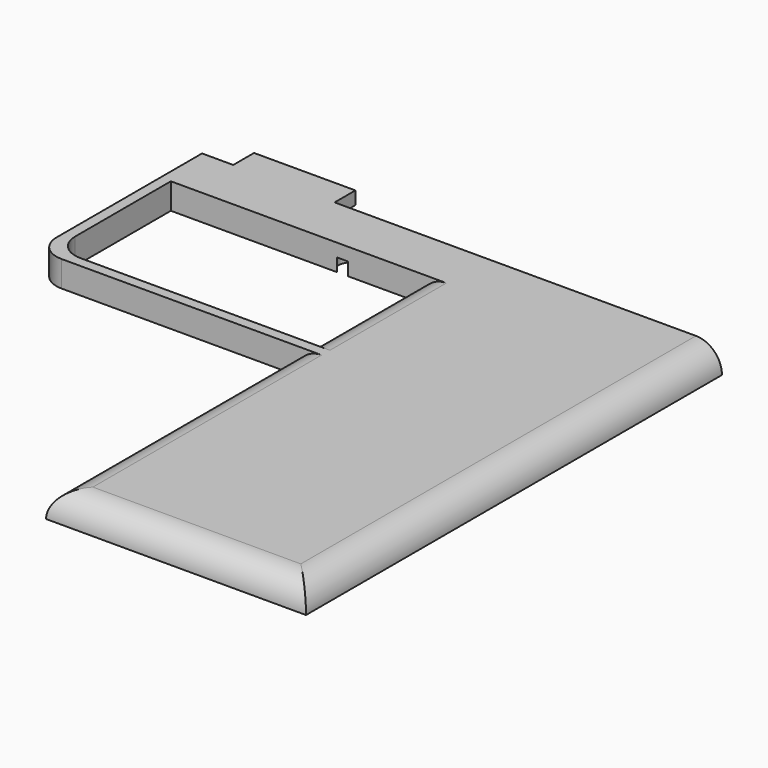
from build123d import *

# Parameters (mm, degrees)
F0_W     = 48
F0_H     = 10
F1_DEPTH = 5
F2_R     = 4.99999
F3_R     = 5
F4_W     = 6
F4_H     = 81
F4_R     = 1.75
F5_DEPTH = 2.5
F6_W     = 19.5
F6_H     = 2.5
F7_DEPTH = 5


# Not quite as in the source:
# - a fillet or chamfer is up to 0.001 mm smaller than in the source, because OpenCascade refuses the exact size


with BuildPart() as f1:
    # F0 (on Top) → F1 (new body)
    with BuildSketch(Plane.XY):
        Polygon((-73, 40), (-73, 50), (-75, 50), (-75, 10), (-25, 10), (-25, 12), (-73, 12), align=None)
        Polygon((25, -50), (25, 50), (-25, 50), (-25, 40), (-25, 12), (-25, 10), (-25, -50), align=None)
        with Locations((-49, 45)):
            Rectangle(F0_W, F0_H)
    extrude(amount=-F1_DEPTH)

    # F2 (radius 5 in the source; OpenCascade refuses exactly that, so slightly less here)
    f2_edges = [f1.edges().sort_by_distance(p)[0] for p in [
        (-25, -20, 0),
        (0, -50, 0),
        (25, 0, 0),
        (-25, 26, 0),
    ]]
    fillet(f2_edges, radius=F2_R)

    # F3
    f3_edges = [f1.edges().sort_by_distance(p)[0] for p in [
        (-73, 12, -2.5),
        (-75, 10, -2.5),
    ]]
    fillet(f3_edges, radius=F3_R)

    # F4 (on face) → F5 (cut)
    with BuildSketch(Plane(origin=(0, 0, -5), x_dir=(1, 0, 0), z_dir=(0, 0, -1))):
        Rectangle(F4_W, F4_H)
        with BuildLine():
            ThreePointArc((-41.0307764064, -40), (-41.1711646096, -43.9211646096), (-37.75, -42))
            ThreePointArc((-37.75, -42), (-38.0788353904, -40.8288353904), (-38.9692235936, -40))
            Line((-38.9692235936, -40), (-41.0307764064, -40))
        make_face()
        with Locations((-50, -48)):
            Circle(F4_R)
        with Locations((-62.5, -45)):
            Circle(F4_R)
        with BuildLine():
            ThreePointArc((-71.25, -42), (-71.7625631329, -40.7625631329), (-73, -40.25))
            ThreePointArc((-73, -40.25), (-74.2374368671, -43.2374368671), (-71.25, -42))
        make_face()
    extrude(amount=-F5_DEPTH, mode=Mode.SUBTRACT)

    # F6 (on face) → F7 (join)
    with BuildSketch(Plane(origin=(0, 50, 0), x_dir=(-1, 0, 0), z_dir=(0, 1, 0))):
        with Locations((59.25, -1.25)):
            Rectangle(F6_W, F6_H)
    extrude(amount=F7_DEPTH)


solid = f1.part
